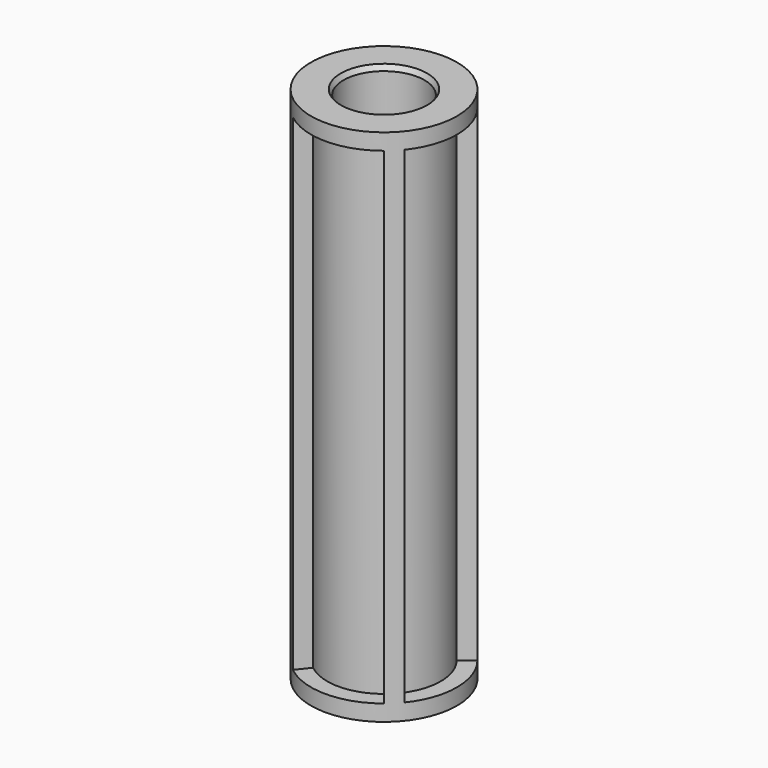
from build123d import *

# Parameters (mm, degrees)
F0_R            = 7.14375
F0_R_2          = 3.96875
F1_DEPTH        = 50.8
F2_SIZE2        = 0.254
F2_SIZE         = 0.508
F6_DEPTH        = 47.625
F6_COPIES_COUNT = 4


# Not quite as in the source:
# - a pattern or mirror of a feature is missing from the dataset's text; its kind, count and spacing are read off the source's solid


with BuildPart() as f1:
    # F0 (on Top) → F1 (new body)
    with BuildSketch(Plane.XY):
        Circle(F0_R)
        Circle(F0_R_2, mode=Mode.SUBTRACT)
    extrude(amount=F1_DEPTH)

    # F2
    f2_edges = [f1.edges().sort_by_distance(p)[0] for p in [
        (-3.96875, 0, 50.8),
        (-3.96875, 0, 0),
    ]]
    f2_side = f1.faces().sort_by_distance((-3.96875, 0, 25.4))[0]
    chamfer(f2_edges, length=F2_SIZE, length2=F2_SIZE2, reference=f2_side)

    # F4 (on offset) → F6 (cut, through all)
    with BuildSketch(Plane(origin=(0, 0, 1.5875), x_dir=(1, 0, 0), z_dir=(0, 0, -1))):
        with BuildLine():
            ThreePointArc((-4.3404758524, -3.4687437838), (-5.55625, 0), (-4.3404758524, 3.4687437838))
            Line((-4.3404758524, 3.4687437838), (-5.5806118102, 4.4598134363))
            ThreePointArc((-5.5806118102, 4.4598134363), (-7.14375, 0), (-5.5806118102, -4.4598134363))
            Line((-5.5806118102, -4.4598134363), (-4.3404758524, -3.4687437838))
        make_face()
    f6 = extrude(amount=-F6_DEPTH, mode=Mode.SUBTRACT)

    # F6_copies: F6 ×4 about axis
    f6_copies_axis = Axis((0, 0, 0), (0, 0, 1))
    for i in range(1, F6_COPIES_COUNT):
        add(f6.rotate(f6_copies_axis, i * 360 / F6_COPIES_COUNT), mode=Mode.SUBTRACT)


solid = f1.part
